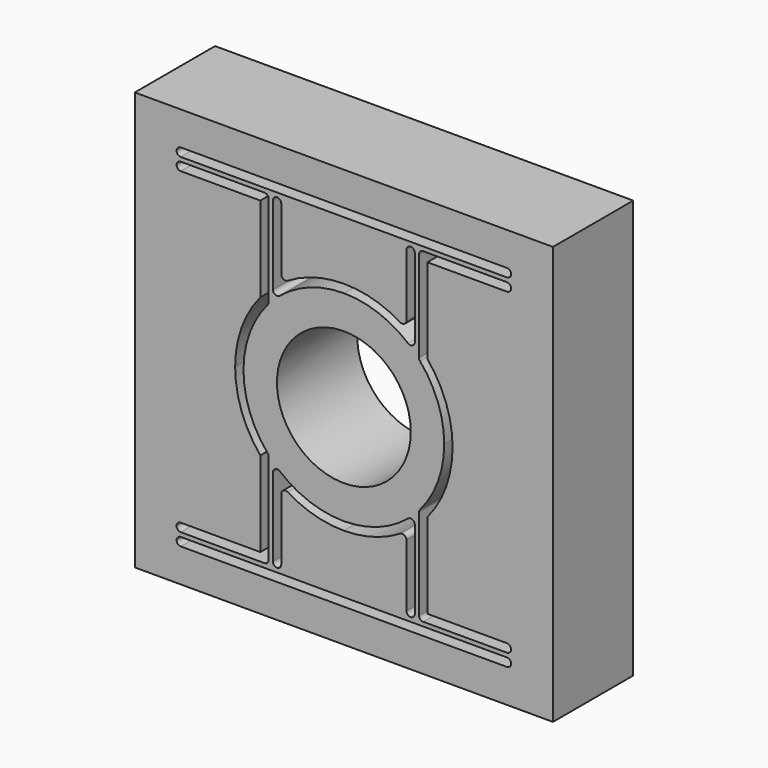
from build123d import *

# Parameters (mm, degrees)
F0_W             = 25
F0_H             = 25
F0_R             = 4
F1_DEPTH         = 3
F2_W             = 10
F2_H             = 0.5
F3_DEPTH         = 6.001
F3_COPIES2_COUNT = 2
F4_R             = 0.24999


# Not quite as in the source:
# - a fillet or chamfer is up to 0.001 mm smaller than in the source, because OpenCascade refuses the exact size
# - a pattern or mirror of a feature is missing from the dataset's text; its kind, count and spacing are read off the source's solid


with BuildPart() as f1:
    # F0 (on Front) → F1 (new body, symmetric)
    with BuildSketch(Plane.XZ):
        Rectangle(F0_W, F0_H)
        Circle(F0_R, mode=Mode.SUBTRACT)
    extrude(amount=F1_DEPTH, both=True)

    # F2 (on face) → F3 (cut, through all)
    with BuildSketch(Plane.XZ.offset(3)):
        with BuildLine():
            ThreePointArc((-4.2426406871, 4.2426406871), (-2.2961005942, 5.5432771951), (0, 6))
            Line((0, 6), (0, 6.5))
            ThreePointArc((0, 6.5), (-1.96297305, 6.1965100504), (-3.7426406871, 5.3143805554))
            Line((-3.7426406871, 5.3143805554), (-3.7426406871, 9.75))
            Line((-3.7426406871, 9.75), (-4.2426406871, 9.75))
            Line((-4.2426406871, 9.75), (-4.2426406871, 4.2426406871))
        make_face()
        with BuildLine():
            Line((-6.5, 0), (-6, 0))
            ThreePointArc((-6, 0), (-5.6105188763, 2.1265177965), (-4.4926406871, 3.9769560793))
            Line((-4.4926406871, 3.9769560793), (-4.4926406871, 9.75))
            Line((-4.4926406871, 9.75), (-10, 9.75))
            Line((-10, 9.75), (-10, 9.25))
            Line((-10, 9.25), (-4.9926406871, 9.25))
            Line((-4.9926406871, 9.25), (-4.9926406871, 4.1621555677))
            ThreePointArc((-4.9926406871, 4.1621555677), (-6.1115531768, 2.2133498971), (-6.5, 0))
        make_face()
        with Locations((-5, 10.25)):
            Rectangle(F2_W, F2_H)
    f3 = extrude(amount=-F3_DEPTH, mode=Mode.SUBTRACT)

    # F3_copies: F3 across plane
    add(f3.mirror(Plane(origin=(0, 0, 0), x_dir=(-1, 0, 0), z_dir=(0, 0, -1))), mode=Mode.SUBTRACT)

    # F3_copies1: F3 across plane
    add(f3.mirror(Plane(origin=(0, 0, 0), x_dir=(0, 0, 1), z_dir=(1, 0, 0))), mode=Mode.SUBTRACT)

    # F3_copies2: F3 ×2 about axis
    f3_copies2_axis = Axis((0, 0, 0), (0, 1, 0))
    for i in range(1, F3_COPIES2_COUNT):
        add(f3.rotate(f3_copies2_axis, i * 360 / F3_COPIES2_COUNT), mode=Mode.SUBTRACT)

    # F4 (radius 0.25 in the source; OpenCascade refuses exactly that, so slightly less here)
    f4_edges = [f1.edges().sort_by_distance(p)[0] for p in [
        (-10, 0, 10),
        (-4.492641, 0, 9.75),
        (-4.492641, 0, 3.976956),
        (-4.242641, 0, 4.242641),
        (-10, 0, 10.5),
        (-4.242641, 0, 9.75),
        (-10, 0, 9.25),
        (-10, 0, 9.75),
        (-3.742641, 0, 9.75),
        (-3.742641, 0, 5.314381),
        (10, 0, 10),
        (10, 0, 10.5),
        (10, 0, 9.25),
        (10, 0, 9.75),
        (4.492641, 0, 9.75),
        (4.492641, 0, 3.976956),
        (4.492641, 0, -3.976956),
        (4.492641, 0, -9.75),
        (10, 0, -9.75),
        (10, 0, -9.25),
        (4.242641, 0, 4.242641),
        (4.242641, 0, 9.75),
        (3.742641, 0, 9.75),
        (3.742641, 0, 5.314381),
        (-10, 0, -9.25),
        (-10, 0, -9.75),
        (-4.492641, 0, -9.75),
        (-4.492641, 0, -3.976956),
        (-3.742641, 0, -9.75),
        (-3.742641, 0, -5.314381),
        (3.742641, 0, -5.314381),
        (3.742641, 0, -9.75),
        (4.242641, 0, -9.75),
        (4.242641, 0, -4.242641),
        (-4.242641, 0, -4.242641),
        (-4.242641, 0, -9.75),
        (10, 0, -10),
        (10, 0, -10.5),
        (-10, 0, -10),
        (-10, 0, -10.5),
    ]]
    fillet(f4_edges, radius=F4_R)


solid = f1.part
